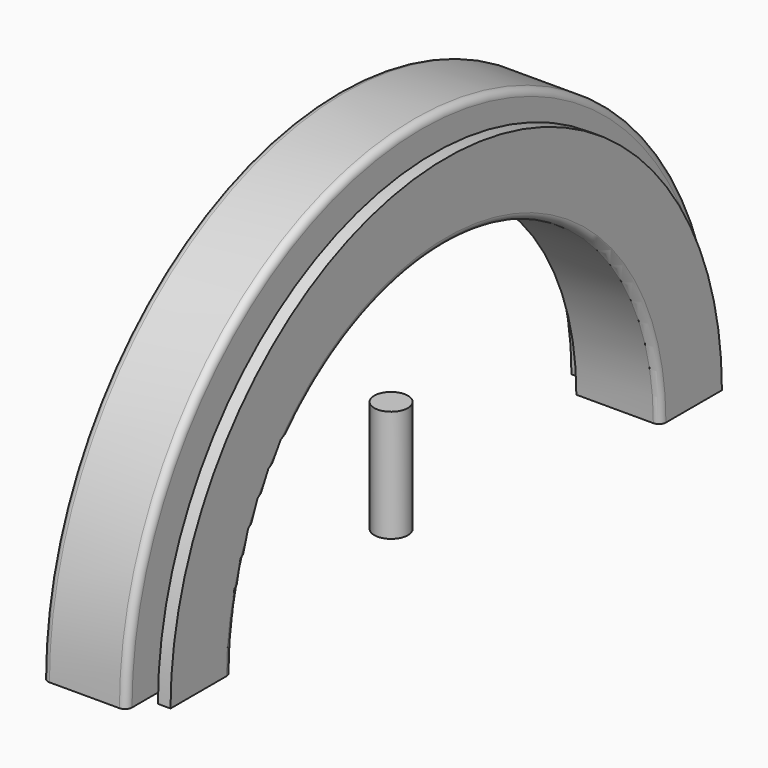
from build123d import *

# Parameters (mm, degrees)
F1_ANGLE = 180
F2_R     = 2.65
F3_DEPTH = 10
F4_R     = 2.4
F5_DEPTH = 16
F6_R     = 1


# Not quite as in the source:
# - a feature names something its author has since deleted; it is built from what else it names


with BuildPart() as f1:
    # F0 (on Top) → F1 (revolve)
    with BuildSketch(Plane.XY):
        Polygon((-7.6431803294, 52.75), (-7.6431803294, 41.75), (-5.8431803294, 41.75), (-5.8431803294, 49.25), (-4.1431803294, 49.25), (-4.1431803294, 38.25), (7.8568196706, 38.25), (7.8568196706, 49.25), (6.0568196706, 49.25), (6.0568196706, 41.75), (4.3568196706, 41.75), (4.3568196706, 52.75), align=None)
    revolve(axis=Axis((-8.8856732473, 0, 0), (1, 0, 0)), revolution_arc=F1_ANGLE)

    # F2 (on Top) → F3 (cut)
    with BuildSketch(Plane.XY):
        with Locations((0, 44.7746068239)):
            Circle(F2_R)
        with Locations((0, -44.7746068239)):
            Circle(F2_R)
    extrude(amount=F3_DEPTH, mode=Mode.SUBTRACT)

    # F6
    f6_edges = [f1.edges().sort_by_distance(p)[0] for p in [
        (7.85682, 0, 38.25),
        (4.35682, 0, 52.75),
        (-7.64318, 0, 52.75),
    ]]
    fillet(f6_edges, radius=F6_R)


with BuildPart() as f5:
    # F4 (on Top) → F5 (new body)
    with BuildSketch(Plane.XY):
        with Locations((-0.019186803, 0)):
            Circle(F4_R)
    extrude(amount=F5_DEPTH)


solid = Compound([f1.part, f5.part])
